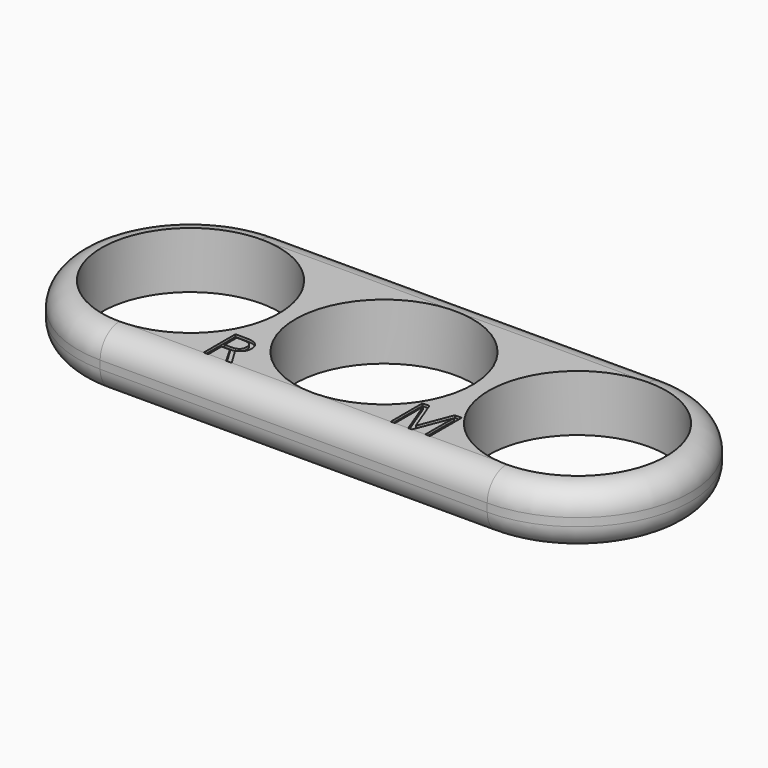
from build123d import *
from build123d import SkipClean  # not in build123d's __all__

# Parameters (mm, degrees)
F0_R         = 11
F1_DEPTH     = 7
F3_R         = 2.99999
F4_R         = 2.99999
F5_TEXT_SIZE = 6.8890318895
F6_DEPTH     = 0.3


# Not quite as in the source:
# - a fillet or chamfer is up to 0.001 mm smaller than in the source, because OpenCascade refuses the exact size
# - Text() gives the source's letters only with a copy of the font that has no kerning and outlines rounded to 1/6400 em; it was checked with that copy


with BuildPart() as f1:
    # F0 (on Top) → F1 (new body)
    with BuildSketch(Plane.XY):
        with BuildLine():
            ThreePointArc((0, -11), (-11, 0), (0, 11))
            Line((0, 11), (0, 14))
            Line((0, 14), (-24, 14))
            ThreePointArc((-24, 14), (-38, 0), (-24, -14))
            Line((-24, -14), (0, -14))
            Line((0, -14), (0, -11))
        make_face()
        with Locations((-24, 0)):
            Circle(F0_R, mode=Mode.SUBTRACT)
    extrude(amount=F1_DEPTH)

    # F2: F1 across plane


with BuildPart() as f1_1:
    add(f1.part, clean=False)
    with SkipClean():  # cleaning this boolean's faces spoils the solid; the shape is the same uncleaned
        add(f1.part.mirror(Plane.YZ), clean=False)

    # F3 (radius 3 in the source; OpenCascade refuses exactly that, so slightly less here)
    f3_edges = [f1_1.edges().sort_by_distance(p)[0] for p in [
        (38, 0, 0),
    ]]
    fillet(f3_edges, radius=F3_R)

    # F4 (radius 3 in the source; OpenCascade refuses exactly that, so slightly less here)
    f4_edges = [f1_1.edges().sort_by_distance(p)[0] for p in [
        (38, 0, 7),
        (-12, 14, 7),
        (12, 14, 7),
        (-38, 0, 7),
        (-12, -14, 7),
        (12, -14, 7),
    ]]
    fillet(f4_edges, radius=F4_R)

    # F5 (on face) → F6 (cut)
    with BuildSketch(Plane.XY.offset(7)):
        with Locations((-14.2320785671, -11)):
            Text('R', F5_TEXT_SIZE, font='Open Sans', text_align=(TextAlign.LEFT, TextAlign.BOTTOM))
        with Locations((8.9580137283, -11)):
            Text('M', F5_TEXT_SIZE, font='Open Sans', text_align=(TextAlign.LEFT, TextAlign.BOTTOM))
    extrude(amount=-F6_DEPTH, mode=Mode.SUBTRACT)


solid = f1_1.part
